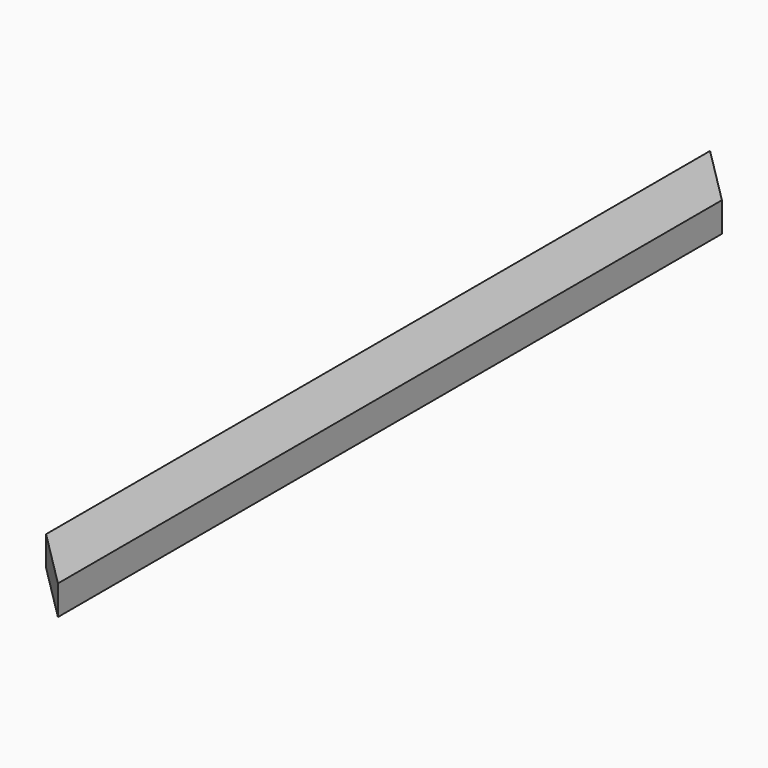
from build123d import *

# Parameters (mm, degrees)
F0_W     = 50.8
F0_H     = 25.4
F1_DEPTH = 762
F2_SIZE  = 50.79999
F3_SIZE  = 50.79999


# Not quite as in the source:
# - a fillet or chamfer is up to 0.001 mm smaller than in the source, because OpenCascade refuses the exact size


with BuildPart() as f1:
    # F0 (on Front) → F1 (new body)
    with BuildSketch(Plane.XZ):
        with Locations((-30.3273661993, 19.0948233087)):
            Rectangle(F0_W, F0_H)
    extrude(amount=F1_DEPTH)

    # F2 (size 50.8 in the source; OpenCascade refuses exactly that, so slightly less here)
    f2_edges = [f1.edges().sort_by_distance(p)[0] for p in [
        (-55.727366, -762, 19.094823),
    ]]
    chamfer(f2_edges, length=F2_SIZE)

    # F3 (size 50.8 in the source; OpenCascade refuses exactly that, so slightly less here)
    f3_edges = [f1.edges().sort_by_distance(p)[0] for p in [
        (-4.927366, 0, 19.094823),
    ]]
    chamfer(f3_edges, length=F3_SIZE)


solid = f1.part
